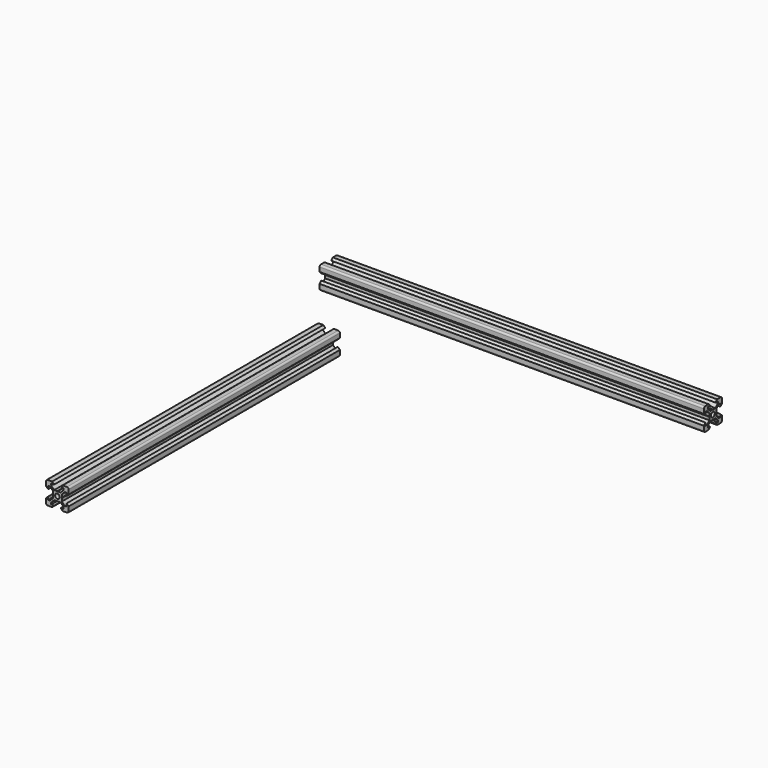
from build123d import *

# Parameters (mm, degrees)
F0_R     = 2.1
F2_DEPTH = 300
F1_R     = 2.1
F3_DEPTH = 340


# Not quite as in the source:
# - ends of sketch curves that miss each other by under 0.0002 mm in the source are joined


with BuildPart() as f2:
    # F0 (on Front) → F2 (new body)
    with BuildSketch(Plane.XZ):
        with BuildLine():
            Line((-4.6400004426, 10.0000019805), (-8.5000014426, 10.0000019805))
            ThreePointArc((-8.5000014426, 10.0000019805), (-9.560661968, 9.5606617987), (-10.0000014426, 8.5000009805))
            Line((-10.0000014426, 8.5000009805), (-10.0000014426, 4.6400009805))
            Line((-10.0000014426, 4.6400009805), (-8.1999994426, 2.8400009805))
            Line((-8.1999994426, 2.8400009805), (-8.1999994426, 5.4993389805))
            Line((-8.1999994426, 5.4993389805), (-6.5600004426, 5.4993389805))
            Line((-6.5600004426, 5.4993389805), (-3.9006604426, 2.8400009805))
            Line((-3.9006604426, 2.8400009805), (-3.9006604426, 0.1999999805))
            Line((-3.9006604426, 0.1999999805), (-3.7006604426, -1.95e-08))
            Line((-3.7006604426, -1.95e-08), (-3.9006604426, -0.2000000195))
            Line((-3.9006604426, -0.2000000195), (-3.9006604426, -2.8400010195))
            Line((-3.9006604426, -2.8400010195), (-6.5600004426, -5.4993410195))
            Line((-6.5600004426, -5.4993410195), (-8.1999994426, -5.4993410195))
            Line((-8.1999994426, -5.4993410195), (-8.1999994426, -2.8400010195))
            Line((-8.1999994426, -2.8400010195), (-10.0000014426, -4.6400010195))
            Line((-10.0000014426, -4.6400010195), (-10.0000014426, -8.5000010195))
            ThreePointArc((-10.0000014426, -8.5000010195), (-9.5606612608, -9.5606615448), (-8.5000014426, -10.0000010195))
            Line((-8.5000014426, -10.0000010195), (-4.6400004426, -10.0000010195))
            Line((-4.6400004426, -10.0000010195), (-2.8400004426, -8.2000000195))
            Line((-2.8400004426, -8.2000000195), (-5.4993404426, -8.2000000195))
            Line((-5.4993404426, -8.2000000195), (-5.4993404426, -6.5600010195))
            Line((-5.4993404426, -6.5600010195), (-2.8400004426, -3.9006610195))
            Line((-2.8400004426, -3.9006610195), (-0.1999994426, -3.9006610195))
            Line((-0.1999994426, -3.9006610195), (5.574e-07, -3.7006610195))
            Line((5.574e-07, -3.7006610195), (0.2000005574, -3.9006610195))
            Line((0.2000005574, -3.9006610195), (2.8399995574, -3.9006610195))
            Line((2.8399995574, -3.9006610195), (5.4993415574, -6.5600010195))
            Line((5.4993415574, -6.5600010195), (5.4993415574, -8.2000000195))
            Line((5.4993415574, -8.2000000195), (2.8399995574, -8.2000000195))
            Line((2.8399995574, -8.2000000195), (4.6399995574, -10.0000010195))
            Line((4.6399995574, -10.0000010195), (8.5000005574, -10.0000010195))
            ThreePointArc((8.5000005574, -10.0000010195), (9.5606607292, -9.5606611913), (10.0000005574, -8.5000010195))
            Line((10.0000005574, -8.5000010195), (10.0000005574, -4.6400010195))
            Line((10.0000005574, -4.6400010195), (8.2000005574, -2.8400010195))
            Line((8.2000005574, -2.8400010195), (8.2000005574, -5.4993410195))
            Line((8.2000005574, -5.4993410195), (6.5600015574, -5.4993410195))
            Line((6.5600015574, -5.4993410195), (3.9006595574, -2.8400010195))
            Line((3.9006595574, -2.8400010195), (3.9006595574, -0.2000000195))
            Line((3.9006595574, -0.2000000195), (3.7006595574, -1.95e-08))
            Line((3.7006595574, -1.95e-08), (3.9006595574, 0.1999999805))
            Line((3.9006595574, 0.1999999805), (3.9006595574, 2.8400009805))
            Line((3.9006595574, 2.8400009805), (6.5600015574, 5.4993389805))
            Line((6.5600015574, 5.4993389805), (8.2000005574, 5.4993389805))
            Line((8.2000005574, 5.4993389805), (8.2000005574, 2.8400009805))
            Line((8.2000005574, 2.8400009805), (10.0000005574, 4.6400009805))
            Line((10.0000005574, 4.6400009805), (10.0000005574, 8.5000019805))
            ThreePointArc((10.0000005574, 8.5000019805), (9.5606607292, 9.5606621523), (8.5000005574, 10.0000019805))
            Line((8.5000005574, 10.0000019805), (4.6399995574, 10.0000019805))
            Line((4.6399995574, 10.0000019805), (2.8399995574, 8.2000019805))
            Line((2.8399995574, 8.2000019805), (5.4993415574, 8.2000019805))
            Line((5.4993415574, 8.2000019805), (5.4993415574, 6.5599989805))
            Line((5.4993415574, 6.5599989805), (2.8399995574, 3.9006609805))
            Line((2.8399995574, 3.9006609805), (0.2000005574, 3.9006609805))
            Line((0.2000005574, 3.9006609805), (5.574e-07, 3.7006609805))
            Line((5.574e-07, 3.7006609805), (-0.1999994426, 3.9006609805))
            Line((-0.1999994426, 3.9006609805), (-2.8400004426, 3.9006609805))
            Line((-2.8400004426, 3.9006609805), (-5.4993404426, 6.5599989805))
            Line((-5.4993404426, 6.5599989805), (-5.4993404426, 8.2000019805))
            Line((-5.4993404426, 8.2000019805), (-2.8400004426, 8.2000019805))
            Line((-2.8400004426, 8.2000019805), (-4.6400004426, 10.0000019805))
        make_face()
        with Locations((5.574e-07, -1.95e-08)):
            Circle(F0_R, mode=Mode.SUBTRACT)
    extrude(amount=F2_DEPTH)


with BuildPart() as f3:
    # F1 (on Right) → F3 (new body)
    with BuildSketch(Plane.YZ):
        with BuildLine():
            Line((-4.5399968378, 62.209959795), (-8.3999978378, 62.209959795))
            ThreePointArc((-8.3999978378, 62.209959795), (-9.4606583632, 61.7706196132), (-9.8999978378, 60.709958795))
            Line((-9.8999978378, 60.709958795), (-9.8999978378, 56.849958795))
            Line((-9.8999978378, 56.849958795), (-8.0999958378, 55.049958795))
            Line((-8.0999958378, 55.049958795), (-8.0999958378, 57.709296795))
            Line((-8.0999958378, 57.709296795), (-6.4599968378, 57.709296795))
            Line((-6.4599968378, 57.709296795), (-3.8006568378, 55.049958795))
            Line((-3.8006568378, 55.049958795), (-3.8006568378, 52.409957795))
            Line((-3.8006568378, 52.409957795), (-3.6006568378, 52.209957795))
            Line((-3.6006568378, 52.209957795), (-3.8006568378, 52.009957795))
            Line((-3.8006568378, 52.009957795), (-3.8006568378, 49.369956795))
            Line((-3.8006568378, 49.369956795), (-6.4599968378, 46.710616795))
            Line((-6.4599968378, 46.710616795), (-8.0999958378, 46.710616795))
            Line((-8.0999958378, 46.710616795), (-8.0999958378, 49.369956795))
            Line((-8.0999958378, 49.369956795), (-9.8999978378, 47.569956795))
            Line((-9.8999978378, 47.569956795), (-9.8999978378, 43.709956795))
            ThreePointArc((-9.8999978378, 43.709956795), (-9.4606576561, 42.6492962696), (-8.3999978378, 42.209956795))
            Line((-8.3999978378, 42.209956795), (-4.5399968378, 42.209956795))
            Line((-4.5399968378, 42.209956795), (-2.7399968378, 44.009957795))
            Line((-2.7399968378, 44.009957795), (-5.3993368378, 44.009957795))
            Line((-5.3993368378, 44.009957795), (-5.3993368378, 45.649956795))
            Line((-5.3993368378, 45.649956795), (-2.7399968378, 48.309296795))
            Line((-2.7399968378, 48.309296795), (-0.0999958378, 48.309296795))
            Line((-0.0999958378, 48.309296795), (0.1000041622, 48.509296795))
            Line((0.1000041622, 48.509296795), (0.3000041622, 48.309296795))
            Line((0.3000041622, 48.309296795), (2.9400031622, 48.309296795))
            Line((2.9400031622, 48.309296795), (5.5993451622, 45.649956795))
            Line((5.5993451622, 45.649956795), (5.5993451622, 44.009957795))
            Line((5.5993451622, 44.009957795), (2.9400031622, 44.009957795))
            Line((2.9400031622, 44.009957795), (4.7400031622, 42.209956795))
            Line((4.7400031622, 42.209956795), (8.6000041622, 42.209956795))
            ThreePointArc((8.6000041622, 42.209956795), (9.6606643339, 42.6492966232), (10.1000041622, 43.709956795))
            Line((10.1000041622, 43.709956795), (10.1000041622, 47.569956795))
            Line((10.1000041622, 47.569956795), (8.3000041622, 49.369956795))
            Line((8.3000041622, 49.369956795), (8.3000041622, 46.710616795))
            Line((8.3000041622, 46.710616795), (6.6600051622, 46.710616795))
            Line((6.6600051622, 46.710616795), (4.0006631622, 49.369956795))
            Line((4.0006631622, 49.369956795), (4.0006631622, 52.009957795))
            Line((4.0006631622, 52.009957795), (3.8006631622, 52.209957795))
            Line((3.8006631622, 52.209957795), (4.0006631622, 52.409957795))
            Line((4.0006631622, 52.409957795), (4.0006631622, 55.049958795))
            Line((4.0006631622, 55.049958795), (6.6600051622, 57.709296795))
            Line((6.6600051622, 57.709296795), (8.3000041622, 57.709296795))
            Line((8.3000041622, 57.709296795), (8.3000041622, 55.049958795))
            Line((8.3000041622, 55.049958795), (10.1000041622, 56.849958795))
            Line((10.1000041622, 56.849958795), (10.1000041622, 60.709959795))
            ThreePointArc((10.1000041622, 60.709959795), (9.6606643339, 61.7706199668), (8.6000041622, 62.209959795))
            Line((8.6000041622, 62.209959795), (4.7400031622, 62.209959795))
            Line((4.7400031622, 62.209959795), (2.9400031622, 60.409959795))
            Line((2.9400031622, 60.409959795), (5.5993451622, 60.409959795))
            Line((5.5993451622, 60.409959795), (5.5993451622, 58.769956795))
            Line((5.5993451622, 58.769956795), (2.9400031622, 56.110618795))
            Line((2.9400031622, 56.110618795), (0.3000041622, 56.110618795))
            Line((0.3000041622, 56.110618795), (0.1000041622, 55.910618795))
            Line((0.1000041622, 55.910618795), (-0.0999958378, 56.110618795))
            Line((-0.0999958378, 56.110618795), (-2.7399968378, 56.110618795))
            Line((-2.7399968378, 56.110618795), (-5.3993368378, 58.769956795))
            Line((-5.3993368378, 58.769956795), (-5.3993368378, 60.409959795))
            Line((-5.3993368378, 60.409959795), (-2.7399968378, 60.409959795))
            Line((-2.7399968378, 60.409959795), (-4.5399968378, 62.209959795))
        make_face()
        with Locations((0.1000041622, 52.209957795)):
            Circle(F1_R, mode=Mode.SUBTRACT)
    extrude(amount=F3_DEPTH)


solid = Compound([f2.part, f3.part])
